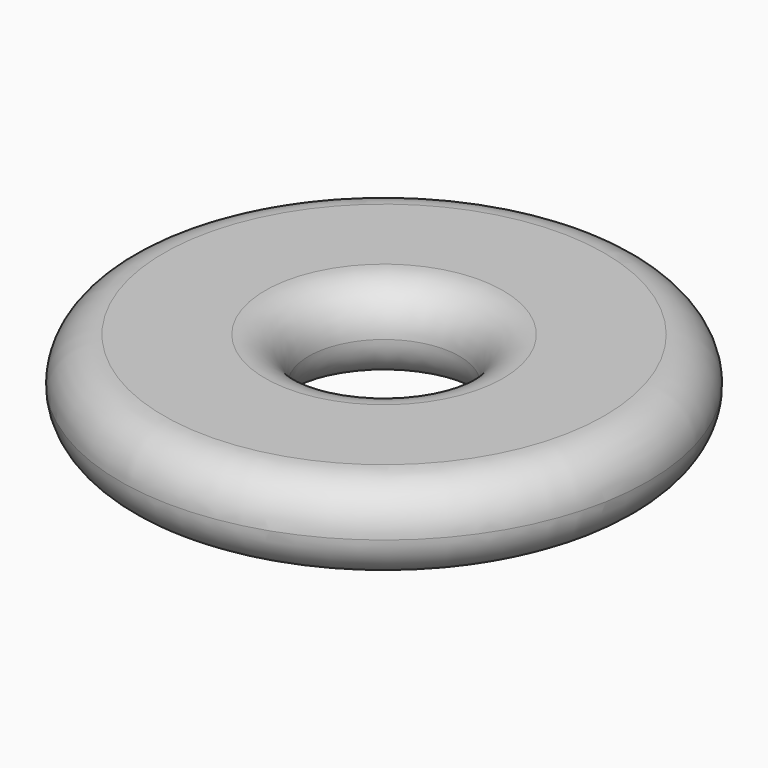
from build123d import *

# Parameters (mm, degrees)
F0_R     = 76.8798317076
F0_R_2   = 21.949412209
F1_DEPTH = 25.4
F2_R     = 12.7
F3_R     = 12.69999
F4_R     = 12.7
F5_R     = 12.69999


# Not quite as in the source:
# - a fillet or chamfer is up to 0.001 mm smaller than in the source, because OpenCascade refuses the exact size


with BuildPart() as f1:
    # F0 (on Top) → F1 (new body)
    with BuildSketch(Plane.XY):
        Circle(F0_R)
        Circle(F0_R_2, mode=Mode.SUBTRACT)
    extrude(amount=F1_DEPTH)

    # F2
    f2_edges = [f1.edges().sort_by_distance(p)[0] for p in [
        (-76.879832, 0, 25.4),
    ]]
    fillet(f2_edges, radius=F2_R)

    # F3 (radius 12.7 in the source; OpenCascade refuses exactly that, so slightly less here)
    f3_edges = [f1.edges().sort_by_distance(p)[0] for p in [
        (-76.879832, 0, 0),
    ]]
    fillet(f3_edges, radius=F3_R)

    # F4
    f4_edges = [f1.edges().sort_by_distance(p)[0] for p in [
        (-21.949412, 0, 25.4),
    ]]
    fillet(f4_edges, radius=F4_R)

    # F5 (radius 12.7 in the source; OpenCascade refuses exactly that, so slightly less here)
    f5_edges = [f1.edges().sort_by_distance(p)[0] for p in [
        (-21.949412, 0, 0),
    ]]
    fillet(f5_edges, radius=F5_R)


solid = f1.part
